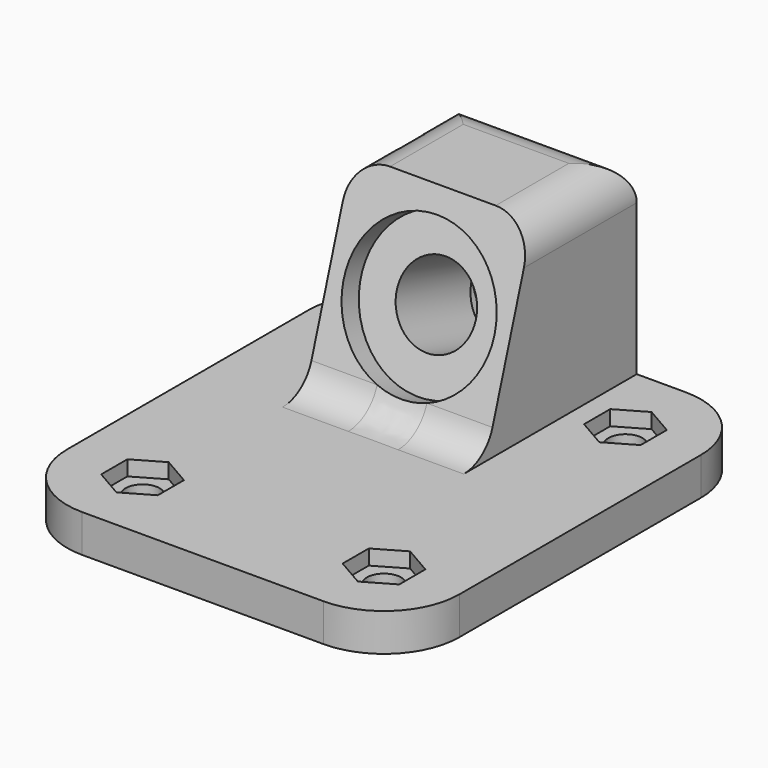
from build123d import *

# Parameters (mm, degrees)
F0_W         = 52
F0_H         = 60
F1_DEPTH     = 5
F2_R         = 10
F3_R         = 2.25
F4_DEPTH     = 25
F6_DEPTH     = 2
F7_W         = 24
F7_H         = 25
F8_DEPTH     = 25
F10_DEPTH    = 40.501
F11_R        = 5.25
F12_DEPTH    = 25.3474527662
F13_R        = 10
F13_R_2      = 5.25
F14_DEPTH    = 3
F16_R        = 10
F17_DEPTH    = 12
F18_DEPTH    = 25.001
F19_F1_R     = 5
F19_T2_DEPTH = 31.5358983849
F19_T4_DEPTH = 28.6534286629
F19_T6_DEPTH = 42.117530278
F19_T8_DEPTH = 49


# Not quite as in the source:
# - a fillet or chamfer that OpenCascade refuses, or shapes differently, is made with other operations: its cross-section is extruded or revolved along the edge and cut away or added


with BuildPart() as f1:
    # F0 (on Top) → F1 (new body)
    with BuildSketch(Plane.XY):
        Rectangle(F0_W, F0_H)
    extrude(amount=F1_DEPTH)

    # F2
    f2_edges = [f1.edges().sort_by_distance(p)[0] for p in [
        (26, -30, 2.5),
        (-26, -30, 2.5),
        (26, 30, 2.5),
        (-26, 30, 2.5),
    ]]
    fillet(f2_edges, radius=F2_R)

    # F3 (on face) → F4 (cut)
    with BuildSketch(Plane.XY.offset(5)):
        with Locations((-16, -20)):
            Circle(F3_R)
        with Locations((16, -20)):
            Circle(F3_R)
        with Locations((-16, 20)):
            Circle(F3_R)
        with Locations((16, 20)):
            Circle(F3_R)
    extrude(amount=-F4_DEPTH, mode=Mode.SUBTRACT)

    # F5 (on face) → F6 (cut)
    with BuildSketch(Plane.XY.offset(5)):
        Polygon((-16, -15.6698729811), (-19.75, -17.8349364905), (-19.75, -22.1650635095), (-16, -24.3301270189), (-12.25, -22.1650635095), (-12.25, -17.8349364905), align=None)
        Polygon((-12.25, 22.1650635095), (-16, 24.3301270189), (-19.75, 22.1650635095), (-19.75, 17.8349364905), (-16, 15.6698729811), (-12.25, 17.8349364905), align=None)
        Polygon((19.75, -17.8349364905), (16, -15.6698729811), (12.25, -17.8349364905), (12.25, -22.1650635095), (16, -24.3301270189), (19.75, -22.1650635095), align=None)
        Polygon((19.75, 22.1650635095), (16, 24.3301270189), (12.25, 22.1650635095), (12.25, 17.8349364905), (16, 15.6698729811), (19.75, 17.8349364905), align=None)
    extrude(amount=-F6_DEPTH, mode=Mode.SUBTRACT)

    # F7 (on face) → F8 (join)
    with BuildSketch(Plane.XY.offset(5)):
        with Locations((-2.5, 17.5)):
            Rectangle(F7_W, F7_H)
    extrude(amount=F8_DEPTH)

    # F9 (on face) → F10 (cut, through all)
    with BuildSketch(Plane(origin=(-14.5, 0, 0), x_dir=(0, -1, 0), z_dir=(-1, 0, 0))):
        Polygon((-12.882469722, 30), (-5, 5), (-5, 30), align=None)
    extrude(amount=-F10_DEPTH, mode=Mode.SUBTRACT)

    # F11 (on face) → F12 (cut, through all)
    with BuildSketch(Plane(origin=(0, 3.1139390198, -0.9818212016), x_dir=(1, 0, 0), z_dir=(0, -0.9537169507, 0.3007057995))):
        with Locations((-2.5, 19.3787278155)):
            Circle(F11_R)
    extrude(amount=-F12_DEPTH, mode=Mode.SUBTRACT)

    # F13 (on face) → F14 (cut)
    with BuildSketch(Plane(origin=(0, 3.1139390198, -0.9818212016), x_dir=(1, 0, 0), z_dir=(0, -0.9537169507, 0.3007057995))):
        with Locations((-2.5, 19.3787278155)):
            Circle(F13_R)
        with Locations((-2.5, 19.3787278155)):
            Circle(F13_R_2, mode=Mode.SUBTRACT)
    extrude(amount=-F14_DEPTH, mode=Mode.SUBTRACT)

    # F16 (on offset) → F17 (cut)
    with BuildSketch(Plane(origin=(0, 29.8180136408, -9.4015835877), x_dir=(1, 0, 0), z_dir=(0, -0.9537169507, 0.3007057995))):
        with Locations((-2.5, 19.3787278155)):
            Circle(F16_R)
    extrude(amount=F17_DEPTH, mode=Mode.SUBTRACT)

    # F5 (on face) → F18 (cut, through all)
    with BuildSketch(Plane.XY.offset(5)):
        Polygon((-16, -15.6698729811), (-19.75, -17.8349364905), (-19.75, -22.1650635095), (-16, -24.3301270189), (-12.25, -22.1650635095), (-12.25, -17.8349364905), align=None)
        Polygon((-12.25, 22.1650635095), (-16, 24.3301270189), (-19.75, 22.1650635095), (-19.75, 17.8349364905), (-16, 15.6698729811), (-12.25, 17.8349364905), align=None)
        Polygon((19.75, -17.8349364905), (16, -15.6698729811), (12.25, -17.8349364905), (12.25, -22.1650635095), (16, -24.3301270189), (19.75, -22.1650635095), align=None)
        Polygon((19.75, 22.1650635095), (16, 24.3301270189), (12.25, 22.1650635095), (12.25, 17.8349364905), (16, 15.6698729811), (19.75, 17.8349364905), align=None)
    extrude(amount=F18_DEPTH, mode=Mode.SUBTRACT)

    # F19: fillet of radius 5 on 5 edges, made by hand

    # F19_f1
    f19_f1_edges = [f1.edges().sort_by_distance(p)[0] for p in [
        (-2.5, 5, 5),
    ]]
    fillet(f19_f1_edges, radius=F19_F1_R)

    # F19_s3 → F19_t2 (cut)
    with BuildSketch(Plane.XZ.offset(-42.5)):
        with BuildLine():
            ThreePointArc((-14.5, 25), (-13.0355339059, 28.5355339059), (-9.5, 30))
            Line((-9.5, 30), (-9.5, 30.1))
            Line((-9.5, 30.1), (-14.6, 30.1))
            Line((-14.6, 30.1), (-14.6, 25))
            Line((-14.6, 25), (-14.5, 25))
        make_face()
    extrude(amount=F19_T2_DEPTH, mode=Mode.SUBTRACT)

    # F19_s5 → F19_t4 (cut)
    with BuildSketch(Plane.XZ.offset(-29.0358983849)):
        with BuildLine():
            ThreePointArc((-14.5, 25), (-13.0355339059, 28.5355339059), (-9.5, 30))
            Line((-9.5, 30), (-9.5, 30.1))
            Line((-9.5, 30.1), (-14.6, 30.1))
            Line((-14.6, 30.1), (-14.6, 25))
            Line((-14.6, 25), (-14.5, 25))
        make_face()
    extrude(amount=F19_T4_DEPTH, mode=Mode.SUBTRACT)

    # F19_s7 → F19_t6 (cut)
    with BuildSketch(Plane.XZ.offset(-42.5)):
        with BuildLine():
            ThreePointArc((9.5, 25), (8.0355339059, 28.5355339059), (4.5, 30))
            Line((4.5, 30), (4.5, 30.1))
            Line((4.5, 30.1), (9.6, 30.1))
            Line((9.6, 30.1), (9.6, 25))
            Line((9.6, 25), (9.5, 25))
        make_face()
    extrude(amount=F19_T6_DEPTH, mode=Mode.SUBTRACT)

    # F19_s9 → F19_t8 (cut)
    with BuildSketch(Plane.YZ.offset(-27)):
        with BuildLine():
            ThreePointArc((30, 25), (28.5355339059, 28.5355339059), (25, 30))
            Line((25, 30), (25, 30.1))
            Line((25, 30.1), (30.1, 30.1))
            Line((30.1, 30.1), (30.1, 25))
            Line((30.1, 25), (30, 25))
        make_face()
    extrude(amount=F19_T8_DEPTH, mode=Mode.SUBTRACT)


solid = f1.part
